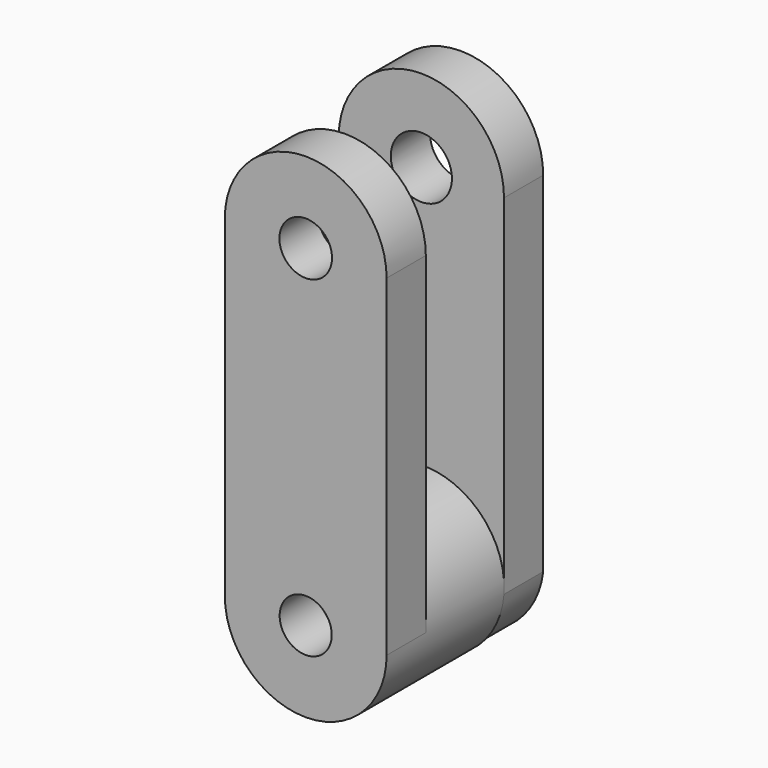
from build123d import *

# Parameters (mm, degrees)
F0_R     = 6.7521335394
F0_R_2   = 6.8163388515
F1_DEPTH = 12.7
F2_R     = 6.7521335394
F3_DEPTH = 25.4
F5_DEPTH = 12.7


# Not quite as in the source:
# - a length typed as a fraction of an inch, garbled in the dataset ("3 / 203.2 mm" for 3/8 in), is restored


with BuildPart() as f1:
    # F0 (on Front) → F1 (new body)
    with BuildSketch(Plane.XZ):
        with BuildLine():
            ThreePointArc((-6.6273338161, 39.4025146961), (-27.5938108098, 60.3689916898), (-48.5602878034, 39.4025146961))
            Line((-48.5602878034, 39.4025146961), (-48.5602878034, -46.63233459))
            ThreePointArc((-48.5602878034, -46.63233459), (-27.5938108098, -67.5988115836), (-6.6273338161, -46.63233459))
            Line((-6.6273338161, -46.63233459), (-6.6273338161, 39.4025146961))
        make_face()
        with Locations((-27.5938108098, -46.63233459)):
            Circle(F0_R, mode=Mode.SUBTRACT)
        with Locations((-27.5938108098, 39.4025146961)):
            Circle(F0_R_2, mode=Mode.SUBTRACT)
    extrude(amount=F1_DEPTH)

    # F2 (on face) → F3 (join)
    with BuildSketch(Plane(origin=(0, 0, 0), x_dir=(-1, 0, 0), z_dir=(0, 1, 0))):
        with BuildLine():
            ThreePointArc((6.6273338161, -46.63233459), (27.5938108098, -67.5988115836), (48.5602878034, -46.63233459))
            ThreePointArc((48.5602878034, -46.63233459), (27.5938108098, -25.6658575963), (6.6273338161, -46.63233459))
        make_face()
        with Locations((27.5938108098, -46.63233459)):
            Circle(F2_R, mode=Mode.SUBTRACT)
    extrude(amount=F3_DEPTH)

    # F4 (on face) → F5 (join)
    with BuildSketch(Plane(origin=(0, 25.4, 0), x_dir=(-1, 0, 0), z_dir=(0, 1, 0))):
        with BuildLine():
            Line((6.6871955224, -45.0491116899), (6.6871955224, -48.21555749))
            Line((6.6871955224, -48.21555749), (20.5757935859, -48.21555749))
            ThreePointArc((20.5757935859, -48.21555749), (20.6464307387, -47.1868562222), (20.8570162136, -46.1774654835))
            ThreePointArc((20.8570162136, -46.1774654835), (25.5313250881, -40.2029131555), (32.8088623121, -42.3434483519))
            ThreePointArc((32.8088623121, -42.3434483519), (34.8864096094, -44.9587614977), (35.6275880547, -48.21555749))
            Line((35.6275880547, -48.21555749), (48.5004260971, -48.21555749))
            ThreePointArc((48.5004260971, -48.21555749), (48.545317032, -47.4245116811), (48.5602878034, -46.63233459))
            ThreePointArc((48.5602878034, -46.63233459), (28.385987901, -25.6808283677), (6.6871955224, -45.0491116899))
        make_face()
        with BuildLine():
            Line((6.6871955224, 42.21310094), (6.6871955224, -45.0491116899))
            ThreePointArc((6.6871955224, -45.0491116899), (28.385987901, -25.6808283677), (48.5602878034, -46.63233459))
            ThreePointArc((48.5602878034, -46.63233459), (48.545317032, -47.4245116811), (48.5004260971, -48.21555749))
            Line((48.5004260971, -48.21555749), (49.5161861181, -48.21555749))
            Line((49.5161861181, -48.21555749), (49.5161861181, 42.21310094))
            Line((49.5161861181, 42.21310094), (36.0246261847, 42.21310094))
            ThreePointArc((36.0246261847, 42.21310094), (28.1016908203, 34.2901655755), (20.1787554558, 42.21310094))
            Line((20.1787554558, 42.21310094), (6.6871955224, 42.21310094))
        make_face()
        with BuildLine():
            Line((20.5757935859, -48.21555749), (6.6871955224, -48.21555749))
            ThreePointArc((6.6871955224, -48.21555749), (17.4268777521, -64.4696352981), (36.8849828604, -65.427740397))
            ThreePointArc((36.8849828604, -65.427740397), (44.9731491209, -58.3605807245), (48.5004260971, -48.21555749))
            Line((48.5004260971, -48.21555749), (35.6275880547, -48.21555749))
            ThreePointArc((35.6275880547, -48.21555749), (28.1016908203, -55.7414547244), (20.5757935859, -48.21555749))
        make_face()
        with BuildLine():
            ThreePointArc((49.5161861181, 42.21310094), (28.1016908203, 63.6275962378), (6.6871955224, 42.21310094))
            Line((6.6871955224, 42.21310094), (20.1787554558, 42.21310094))
            ThreePointArc((20.1787554558, 42.21310094), (28.1016908203, 50.1360363044), (36.0246261847, 42.21310094))
            Line((36.0246261847, 42.21310094), (49.5161861181, 42.21310094))
        make_face()
    extrude(amount=F5_DEPTH)


solid = f1.part
